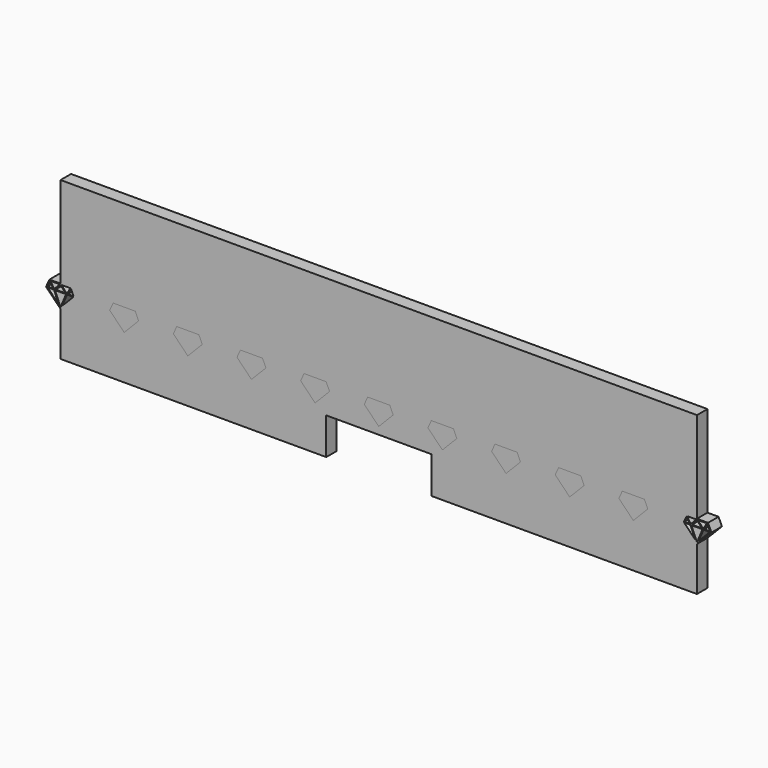
from build123d import *

# Parameters (mm, degrees)
F2_DEPTH = 1.6
F5_DEPTH = 25


# Not quite as in the source:
# - a feature of the source that left no trace in its solid (it failed there, or was rolled back) is left out
# - a feature names something its author has since deleted; it is built from what else it names


with BuildPart() as f2:
    # F0 (on Front) → F2 (new body)
    with BuildSketch(Plane.XZ):
        Polygon((-27.5092766582, 112.0762870512), (0, 83.9119844419), (27.5092766582, 112.0762870512), (21.0788567191, 126.3461877986), (0, 126.3459026814), (-21.0788567191, 126.3461877986), align=None)
        Polygon((-24.595520188, 111.955450038), (-12.439796289, 111.955450038), (-3.5350198746, 90.3934761882), align=None, mode=Mode.SUBTRACT)
        Polygon((10.5240828187, 111.955450038), (0, 86.5410715342), (-10.5240828187, 111.955450038), (0, 111.955450038), align=None, mode=Mode.SUBTRACT)
        Polygon((24.595520188, 111.955450038), (3.5350198746, 90.3934761882), (12.439796289, 111.955450038), align=None, mode=Mode.SUBTRACT)
        Polygon((-19.8720569611, 124.1561621428), (-13.9740581512, 113.2946610451), (-24.7665558411, 113.2946610451), align=None, mode=Mode.SUBTRACT)
        Polygon((-18.6457509995, 124.6817186475), (-1.7468536503, 124.6817186475), (-12.1264214497, 113.0322592129), align=None, mode=Mode.SUBTRACT)
        Polygon((-9.4357720005, 113.2946610451), (0, 123.8848556735), (9.4357720005, 113.2946610451), (0, 113.2946610451), align=None, mode=Mode.SUBTRACT)
        Polygon((12.1264214497, 113.0322592129), (1.7468536503, 124.6817186475), (18.6457509995, 124.6817186475), align=None, mode=Mode.SUBTRACT)
        Polygon((13.9740581512, 113.2946610451), (19.8720569611, 124.1561621428), (24.7665558411, 113.2946610451), align=None, mode=Mode.SUBTRACT)
    extrude(amount=-F2_DEPTH)


with BuildPart() as f2b:
    # F0 (on Front) → F2, piece 2 (new body)
    with BuildSketch(Plane.XZ):
        Polygon((-1069.7211432809, 126.3461877986), (-1090.8, 126.3459026814), (-1111.8788567191, 126.3461877986), (-1118.3092766582, 112.0762870511), (-1090.8, 83.9119844419), (-1063.2907233418, 112.0762870512), align=None)
        Polygon((-1115.395520188, 111.955450038), (-1103.239796289, 111.955450038), (-1094.3350198746, 90.3934761882), align=None, mode=Mode.SUBTRACT)
        Polygon((-1080.2759171813, 111.955450038), (-1090.8, 86.5410715342), (-1101.3240828187, 111.955450038), (-1090.8, 111.955450038), align=None, mode=Mode.SUBTRACT)
        Polygon((-1066.204479812, 111.955450038), (-1087.2649801254, 90.3934761882), (-1078.360203711, 111.955450038), align=None, mode=Mode.SUBTRACT)
        Polygon((-1110.6720569611, 124.1561621428), (-1104.7740581512, 113.2946610451), (-1115.5665558411, 113.2946610451), align=None, mode=Mode.SUBTRACT)
        Polygon((-1109.4457509995, 124.6817186475), (-1092.5468536503, 124.6817186475), (-1102.9264214497, 113.0322592129), align=None, mode=Mode.SUBTRACT)
        Polygon((-1100.2357720005, 113.2946610451), (-1090.8, 123.8848556735), (-1081.3642279995, 113.2946610451), (-1090.8, 113.2946610451), align=None, mode=Mode.SUBTRACT)
        Polygon((-1078.6735785503, 113.0322592129), (-1089.0531463497, 124.6817186475), (-1072.1542490005, 124.6817186475), align=None, mode=Mode.SUBTRACT)
        Polygon((-1076.8259418488, 113.2946610451), (-1070.9279430389, 124.1561621428), (-1066.0334441589, 113.2946610451), align=None, mode=Mode.SUBTRACT)
        Polygon((-1081.3642279995, 113.2946610451), (-1090.8, 123.8848556735), (-1100.2357720005, 113.2946610451), (-1090.8, 113.2946610451), align=None)
        Polygon((-1102.9264214497, 113.0322592129), (-1092.5468536503, 124.6817186475), (-1109.4457509995, 124.6817186475), align=None)
        Polygon((-1072.1542490005, 124.6817186475), (-1089.0531463497, 124.6817186475), (-1078.6735785503, 113.0322592129), align=None)
        Polygon((-1066.0334441589, 113.2946610451), (-1070.9279430389, 124.1561621428), (-1076.8259418488, 113.2946610451), align=None)
        Polygon((-1078.360203711, 111.955450038), (-1087.2649801254, 90.3934761882), (-1066.204479812, 111.955450038), align=None)
        Polygon((-1101.3240828187, 111.955450038), (-1090.8, 86.5410715342), (-1080.2759171813, 111.955450038), (-1090.8, 111.955450038), align=None)
        Polygon((-1094.3350198746, 90.3934761882), (-1103.239796289, 111.955450038), (-1115.395520188, 111.955450038), align=None)
        Polygon((-1115.5665558411, 113.2946610451), (-1104.7740581512, 113.2946610451), (-1110.6720569611, 124.1561621428), align=None)
    extrude(amount=-F2_DEPTH)


with BuildPart() as f2c:
    # F0 (on Front) → F2, piece 3 (new body)
    with BuildSketch(Plane.XZ):
        Polygon((-948.5211432809, 126.3461877986), (-969.6, 126.3459026814), (-990.6788567191, 126.3461877986), (-997.1092766582, 112.0762870511), (-969.6, 83.9119844419), (-942.0907233418, 112.0762870512), align=None)
        Polygon((-994.195520188, 111.955450038), (-982.039796289, 111.955450038), (-973.1350198746, 90.3934761882), align=None, mode=Mode.SUBTRACT)
        Polygon((-959.0759171813, 111.955450038), (-969.6, 86.5410715342), (-980.1240828187, 111.955450038), (-969.6, 111.955450038), align=None, mode=Mode.SUBTRACT)
        Polygon((-945.004479812, 111.955450038), (-966.0649801254, 90.3934761882), (-957.160203711, 111.955450038), align=None, mode=Mode.SUBTRACT)
        Polygon((-989.4720569611, 124.1561621428), (-983.5740581512, 113.2946610451), (-994.3665558411, 113.2946610451), align=None, mode=Mode.SUBTRACT)
        Polygon((-988.2457509995, 124.6817186475), (-971.3468536503, 124.6817186475), (-981.7264214497, 113.0322592129), align=None, mode=Mode.SUBTRACT)
        Polygon((-979.0357720005, 113.2946610451), (-969.6, 123.8848556735), (-960.1642279995, 113.2946610451), (-969.6, 113.2946610451), align=None, mode=Mode.SUBTRACT)
        Polygon((-957.4735785503, 113.0322592129), (-967.8531463497, 124.6817186475), (-950.9542490005, 124.6817186475), align=None, mode=Mode.SUBTRACT)
        Polygon((-955.6259418488, 113.2946610451), (-949.7279430389, 124.1561621428), (-944.8334441589, 113.2946610451), align=None, mode=Mode.SUBTRACT)
        Polygon((-960.1642279995, 113.2946610451), (-969.6, 123.8848556735), (-979.0357720005, 113.2946610451), (-969.6, 113.2946610451), align=None)
        Polygon((-981.7264214497, 113.0322592129), (-971.3468536503, 124.6817186475), (-988.2457509995, 124.6817186475), align=None)
        Polygon((-950.9542490005, 124.6817186475), (-967.8531463497, 124.6817186475), (-957.4735785503, 113.0322592129), align=None)
        Polygon((-944.8334441589, 113.2946610451), (-949.7279430389, 124.1561621428), (-955.6259418488, 113.2946610451), align=None)
        Polygon((-957.160203711, 111.955450038), (-966.0649801254, 90.3934761882), (-945.004479812, 111.955450038), align=None)
        Polygon((-980.1240828187, 111.955450038), (-969.6, 86.5410715342), (-959.0759171813, 111.955450038), (-969.6, 111.955450038), align=None)
        Polygon((-973.1350198746, 90.3934761882), (-982.039796289, 111.955450038), (-994.195520188, 111.955450038), align=None)
        Polygon((-994.3665558411, 113.2946610451), (-983.5740581512, 113.2946610451), (-989.4720569611, 124.1561621428), align=None)
    extrude(amount=-F2_DEPTH)


with BuildPart() as f2d:
    # F0 (on Front) → F2, piece 4 (new body)
    with BuildSketch(Plane.XZ):
        Polygon((-827.3211432809, 126.3461877986), (-848.4, 126.3459026814), (-869.4788567191, 126.3461877986), (-875.9092766582, 112.0762870511), (-848.4, 83.9119844419), (-820.8907233418, 112.0762870512), align=None)
        Polygon((-837.8759171813, 111.955450038), (-848.4, 86.5410715342), (-858.9240828187, 111.955450038), (-848.4, 111.955450038), align=None, mode=Mode.SUBTRACT)
        Polygon((-872.995520188, 111.955450038), (-860.839796289, 111.955450038), (-851.9350198746, 90.3934761882), align=None, mode=Mode.SUBTRACT)
        Polygon((-823.804479812, 111.955450038), (-844.8649801254, 90.3934761882), (-835.960203711, 111.955450038), align=None, mode=Mode.SUBTRACT)
        Polygon((-868.2720569611, 124.1561621428), (-862.3740581512, 113.2946610451), (-873.1665558411, 113.2946610451), align=None, mode=Mode.SUBTRACT)
        Polygon((-867.0457509995, 124.6817186475), (-850.1468536503, 124.6817186475), (-860.5264214497, 113.0322592129), align=None, mode=Mode.SUBTRACT)
        Polygon((-857.8357720005, 113.2946610451), (-848.4, 123.8848556735), (-838.9642279995, 113.2946610451), (-848.4, 113.2946610451), align=None, mode=Mode.SUBTRACT)
        Polygon((-836.2735785503, 113.0322592129), (-846.6531463497, 124.6817186475), (-829.7542490005, 124.6817186475), align=None, mode=Mode.SUBTRACT)
        Polygon((-838.9642279995, 113.2946610451), (-848.4, 123.8848556735), (-857.8357720005, 113.2946610451), (-848.4, 113.2946610451), align=None)
        Polygon((-860.5264214497, 113.0322592129), (-850.1468536503, 124.6817186475), (-867.0457509995, 124.6817186475), align=None)
        Polygon((-829.7542490005, 124.6817186475), (-846.6531463497, 124.6817186475), (-836.2735785503, 113.0322592129), align=None)
        Polygon((-835.960203711, 111.955450038), (-844.8649801254, 90.3934761882), (-823.804479812, 111.955450038), align=None)
        Polygon((-858.9240828187, 111.955450038), (-848.4, 86.5410715342), (-837.8759171813, 111.955450038), (-848.4, 111.955450038), align=None)
        Polygon((-851.9350198746, 90.3934761882), (-860.839796289, 111.955450038), (-872.995520188, 111.955450038), align=None)
        Polygon((-873.1665558411, 113.2946610451), (-862.3740581512, 113.2946610451), (-868.2720569611, 124.1561621428), align=None)
    extrude(amount=-F2_DEPTH)


with BuildPart() as f2e:
    # F0 (on Front) → F2, piece 5 (new body)
    with BuildSketch(Plane.XZ):
        Polygon((-706.1211432809, 126.3461877986), (-727.2, 126.3459026814), (-748.2788567191, 126.3461877986), (-754.7092766582, 112.0762870511), (-727.2, 83.9119844419), (-699.6907233418, 112.0762870512), align=None)
        Polygon((-716.6759171813, 111.955450038), (-727.2, 86.5410715342), (-737.7240828187, 111.955450038), (-727.2, 111.955450038), align=None, mode=Mode.SUBTRACT)
        Polygon((-751.795520188, 111.955450038), (-739.639796289, 111.955450038), (-730.7350198746, 90.3934761882), align=None, mode=Mode.SUBTRACT)
        Polygon((-702.604479812, 111.955450038), (-723.6649801254, 90.3934761882), (-714.760203711, 111.955450038), align=None, mode=Mode.SUBTRACT)
        Polygon((-747.0720569611, 124.1561621428), (-741.1740581512, 113.2946610451), (-751.9665558411, 113.2946610451), align=None, mode=Mode.SUBTRACT)
        Polygon((-745.8457509995, 124.6817186475), (-728.9468536503, 124.6817186475), (-739.3264214497, 113.0322592129), align=None, mode=Mode.SUBTRACT)
        Polygon((-736.6357720005, 113.2946610451), (-727.2, 123.8848556735), (-717.7642279995, 113.2946610451), (-727.2, 113.2946610451), align=None, mode=Mode.SUBTRACT)
        Polygon((-715.0735785503, 113.0322592129), (-725.4531463497, 124.6817186475), (-708.5542490005, 124.6817186475), align=None, mode=Mode.SUBTRACT)
        Polygon((-717.7642279995, 113.2946610451), (-727.2, 123.8848556735), (-736.6357720005, 113.2946610451), (-727.2, 113.2946610451), align=None)
        Polygon((-739.3264214497, 113.0322592129), (-728.9468536503, 124.6817186475), (-745.8457509995, 124.6817186475), align=None)
        Polygon((-708.5542490005, 124.6817186475), (-725.4531463497, 124.6817186475), (-715.0735785503, 113.0322592129), align=None)
        Polygon((-714.760203711, 111.955450038), (-723.6649801254, 90.3934761882), (-702.604479812, 111.955450038), align=None)
        Polygon((-737.7240828187, 111.955450038), (-727.2, 86.5410715342), (-716.6759171813, 111.955450038), (-727.2, 111.955450038), align=None)
        Polygon((-730.7350198746, 90.3934761882), (-739.639796289, 111.955450038), (-751.795520188, 111.955450038), align=None)
        Polygon((-751.9665558411, 113.2946610451), (-741.1740581512, 113.2946610451), (-747.0720569611, 124.1561621428), align=None)
    extrude(amount=-F2_DEPTH)


with BuildPart() as f2f:
    # F0 (on Front) → F2, piece 6 (new body)
    with BuildSketch(Plane.XZ):
        Polygon((-584.9211432809, 126.3461877986), (-606, 126.3459026814), (-627.0788567191, 126.3461877986), (-633.5092766582, 112.0762870511), (-606, 83.9119844419), (-578.4907233418, 112.0762870512), align=None)
        Polygon((-630.595520188, 111.955450038), (-618.439796289, 111.955450038), (-609.5350198746, 90.3934761882), align=None, mode=Mode.SUBTRACT)
        Polygon((-625.8720569611, 124.1561621428), (-619.9740581512, 113.2946610451), (-630.7665558411, 113.2946610451), align=None, mode=Mode.SUBTRACT)
        Polygon((-624.6457509995, 124.6817186475), (-607.7468536503, 124.6817186475), (-618.1264214497, 113.0322592129), align=None, mode=Mode.SUBTRACT)
        Polygon((-595.4759171813, 111.955450038), (-606, 86.5410715342), (-616.5240828187, 111.955450038), (-606, 111.955450038), align=None, mode=Mode.SUBTRACT)
        Polygon((-581.404479812, 111.955450038), (-602.4649801254, 90.3934761882), (-593.560203711, 111.955450038), align=None, mode=Mode.SUBTRACT)
        Polygon((-615.4357720005, 113.2946610451), (-606, 123.8848556735), (-596.5642279995, 113.2946610451), (-606, 113.2946610451), align=None, mode=Mode.SUBTRACT)
        Polygon((-593.8735785503, 113.0322592129), (-604.2531463497, 124.6817186475), (-587.3542490005, 124.6817186475), align=None, mode=Mode.SUBTRACT)
        Polygon((-596.5642279995, 113.2946610451), (-606, 123.8848556735), (-615.4357720005, 113.2946610451), (-606, 113.2946610451), align=None)
        Polygon((-618.1264214497, 113.0322592129), (-607.7468536503, 124.6817186475), (-624.6457509995, 124.6817186475), align=None)
        Polygon((-587.3542490005, 124.6817186475), (-604.2531463497, 124.6817186475), (-593.8735785503, 113.0322592129), align=None)
        Polygon((-593.560203711, 111.955450038), (-602.4649801254, 90.3934761882), (-581.404479812, 111.955450038), align=None)
        Polygon((-616.5240828187, 111.955450038), (-606, 86.5410715342), (-595.4759171813, 111.955450038), (-606, 111.955450038), align=None)
        Polygon((-609.5350198746, 90.3934761882), (-618.439796289, 111.955450038), (-630.595520188, 111.955450038), align=None)
        Polygon((-630.7665558411, 113.2946610451), (-619.9740581512, 113.2946610451), (-625.8720569611, 124.1561621428), align=None)
    extrude(amount=-F2_DEPTH)


with BuildPart() as f2g:
    # F0 (on Front) → F2, piece 7 (new body)
    with BuildSketch(Plane.XZ):
        Polygon((-463.7211432809, 126.3461877986), (-484.8, 126.3459026814), (-505.8788567191, 126.3461877986), (-512.3092766582, 112.0762870511), (-484.8, 83.9119844419), (-457.2907233418, 112.0762870512), align=None)
        Polygon((-509.395520188, 111.955450038), (-497.239796289, 111.955450038), (-488.3350198746, 90.3934761882), align=None, mode=Mode.SUBTRACT)
        Polygon((-474.2759171813, 111.955450038), (-484.8, 86.5410715342), (-495.3240828187, 111.955450038), (-484.8, 111.955450038), align=None, mode=Mode.SUBTRACT)
        Polygon((-460.204479812, 111.955450038), (-481.2649801254, 90.3934761882), (-472.360203711, 111.955450038), align=None, mode=Mode.SUBTRACT)
        Polygon((-504.6720569611, 124.1561621428), (-498.7740581512, 113.2946610451), (-509.5665558411, 113.2946610451), align=None, mode=Mode.SUBTRACT)
        Polygon((-503.4457509995, 124.6817186475), (-486.5468536503, 124.6817186475), (-496.9264214497, 113.0322592129), align=None, mode=Mode.SUBTRACT)
        Polygon((-494.2357720005, 113.2946610451), (-484.8, 123.8848556735), (-475.3642279995, 113.2946610451), (-484.8, 113.2946610451), align=None, mode=Mode.SUBTRACT)
        Polygon((-472.6735785503, 113.0322592129), (-483.0531463497, 124.6817186475), (-466.1542490005, 124.6817186475), align=None, mode=Mode.SUBTRACT)
        Polygon((-475.3642279995, 113.2946610451), (-484.8, 123.8848556735), (-494.2357720005, 113.2946610451), (-484.8, 113.2946610451), align=None)
        Polygon((-496.9264214497, 113.0322592129), (-486.5468536503, 124.6817186475), (-503.4457509995, 124.6817186475), align=None)
        Polygon((-466.1542490005, 124.6817186475), (-483.0531463497, 124.6817186475), (-472.6735785503, 113.0322592129), align=None)
        Polygon((-472.360203711, 111.955450038), (-481.2649801254, 90.3934761882), (-460.204479812, 111.955450038), align=None)
        Polygon((-495.3240828187, 111.955450038), (-484.8, 86.5410715342), (-474.2759171813, 111.955450038), (-484.8, 111.955450038), align=None)
        Polygon((-488.3350198746, 90.3934761882), (-497.239796289, 111.955450038), (-509.395520188, 111.955450038), align=None)
        Polygon((-509.5665558411, 113.2946610451), (-498.7740581512, 113.2946610451), (-504.6720569611, 124.1561621428), align=None)
    extrude(amount=-F2_DEPTH)


with BuildPart() as f2h:
    # F0 (on Front) → F2, piece 8 (new body)
    with BuildSketch(Plane.XZ):
        Polygon((-342.5211432809, 126.3461877986), (-363.6, 126.3459026814), (-384.6788567191, 126.3461877986), (-391.1092766582, 112.0762870511), (-363.6, 83.9119844419), (-336.0907233418, 112.0762870512), align=None)
        Polygon((-388.195520188, 111.955450038), (-376.039796289, 111.955450038), (-367.1350198746, 90.3934761882), align=None, mode=Mode.SUBTRACT)
        Polygon((-353.0759171813, 111.955450038), (-363.6, 86.5410715342), (-374.1240828187, 111.955450038), (-363.6, 111.955450038), align=None, mode=Mode.SUBTRACT)
        Polygon((-339.004479812, 111.955450038), (-360.0649801254, 90.3934761882), (-351.160203711, 111.955450038), align=None, mode=Mode.SUBTRACT)
        Polygon((-383.4720569611, 124.1561621428), (-377.5740581512, 113.2946610451), (-388.3665558411, 113.2946610451), align=None, mode=Mode.SUBTRACT)
        Polygon((-382.2457509995, 124.6817186475), (-365.3468536503, 124.6817186475), (-375.7264214497, 113.0322592129), align=None, mode=Mode.SUBTRACT)
        Polygon((-373.0357720005, 113.2946610451), (-363.6, 123.8848556735), (-354.1642279995, 113.2946610451), (-363.6, 113.2946610451), align=None, mode=Mode.SUBTRACT)
        Polygon((-351.4735785503, 113.0322592129), (-361.8531463497, 124.6817186475), (-344.9542490005, 124.6817186475), align=None, mode=Mode.SUBTRACT)
        Polygon((-354.1642279995, 113.2946610451), (-363.6, 123.8848556735), (-373.0357720005, 113.2946610451), (-363.6, 113.2946610451), align=None)
        Polygon((-375.7264214497, 113.0322592129), (-365.3468536503, 124.6817186475), (-382.2457509995, 124.6817186475), align=None)
        Polygon((-344.9542490005, 124.6817186475), (-361.8531463497, 124.6817186475), (-351.4735785503, 113.0322592129), align=None)
        Polygon((-351.160203711, 111.955450038), (-360.0649801254, 90.3934761882), (-339.004479812, 111.955450038), align=None)
        Polygon((-374.1240828187, 111.955450038), (-363.6, 86.5410715342), (-353.0759171813, 111.955450038), (-363.6, 111.955450038), align=None)
        Polygon((-367.1350198746, 90.3934761882), (-376.039796289, 111.955450038), (-388.195520188, 111.955450038), align=None)
        Polygon((-388.3665558411, 113.2946610451), (-377.5740581512, 113.2946610451), (-383.4720569611, 124.1561621428), align=None)
    extrude(amount=-F2_DEPTH)


with BuildPart() as f2i:
    # F0 (on Front) → F2, piece 9 (new body)
    with BuildSketch(Plane.XZ):
        Polygon((-221.3211432809, 126.3461877986), (-242.4, 126.3459026814), (-263.4788567191, 126.3461877986), (-269.9092766582, 112.0762870511), (-242.4, 83.9119844419), (-214.8907233418, 112.0762870512), align=None)
        Polygon((-266.995520188, 111.955450038), (-254.839796289, 111.955450038), (-245.9350198746, 90.3934761882), align=None, mode=Mode.SUBTRACT)
        Polygon((-231.8759171813, 111.955450038), (-242.4, 86.5410715342), (-252.9240828187, 111.955450038), (-242.4, 111.955450038), align=None, mode=Mode.SUBTRACT)
        Polygon((-217.804479812, 111.955450038), (-238.8649801254, 90.3934761882), (-229.960203711, 111.955450038), align=None, mode=Mode.SUBTRACT)
        Polygon((-262.2720569611, 124.1561621428), (-256.3740581512, 113.2946610451), (-267.1665558411, 113.2946610451), align=None, mode=Mode.SUBTRACT)
        Polygon((-261.0457509995, 124.6817186475), (-244.1468536503, 124.6817186475), (-254.5264214497, 113.0322592129), align=None, mode=Mode.SUBTRACT)
        Polygon((-251.8357720005, 113.2946610451), (-242.4, 123.8848556735), (-232.9642279995, 113.2946610451), (-242.4, 113.2946610451), align=None, mode=Mode.SUBTRACT)
        Polygon((-230.2735785503, 113.0322592129), (-240.6531463497, 124.6817186475), (-223.7542490005, 124.6817186475), align=None, mode=Mode.SUBTRACT)
        Polygon((-232.9642279995, 113.2946610451), (-242.4, 123.8848556735), (-251.8357720005, 113.2946610451), (-242.4, 113.2946610451), align=None)
        Polygon((-254.5264214497, 113.0322592129), (-244.1468536503, 124.6817186475), (-261.0457509995, 124.6817186475), align=None)
        Polygon((-223.7542490005, 124.6817186475), (-240.6531463497, 124.6817186475), (-230.2735785503, 113.0322592129), align=None)
        Polygon((-229.960203711, 111.955450038), (-238.8649801254, 90.3934761882), (-217.804479812, 111.955450038), align=None)
        Polygon((-252.9240828187, 111.955450038), (-242.4, 86.5410715342), (-231.8759171813, 111.955450038), (-242.4, 111.955450038), align=None)
        Polygon((-245.9350198746, 90.3934761882), (-254.839796289, 111.955450038), (-266.995520188, 111.955450038), align=None)
        Polygon((-267.1665558411, 113.2946610451), (-256.3740581512, 113.2946610451), (-262.2720569611, 124.1561621428), align=None)
    extrude(amount=-F2_DEPTH)


with BuildPart() as f2j:
    # F0 (on Front) → F2, piece 10 (new body)
    with BuildSketch(Plane.XZ):
        Polygon((-100.1211432809, 126.3461877986), (-121.2, 126.3459026814), (-142.2788567191, 126.3461877986), (-148.7092766582, 112.0762870511), (-121.2, 83.9119844419), (-93.6907233418, 112.0762870512), align=None)
        Polygon((-145.795520188, 111.955450038), (-133.639796289, 111.955450038), (-124.7350198746, 90.3934761882), align=None, mode=Mode.SUBTRACT)
        Polygon((-110.6759171813, 111.955450038), (-121.2, 86.5410715342), (-131.7240828187, 111.955450038), (-121.2, 111.955450038), align=None, mode=Mode.SUBTRACT)
        Polygon((-96.604479812, 111.955450038), (-117.6649801254, 90.3934761882), (-108.760203711, 111.955450038), align=None, mode=Mode.SUBTRACT)
        Polygon((-141.0720569611, 124.1561621428), (-135.1740581512, 113.2946610451), (-145.9665558411, 113.2946610451), align=None, mode=Mode.SUBTRACT)
        Polygon((-139.8457509995, 124.6817186475), (-122.9468536503, 124.6817186475), (-133.3264214497, 113.0322592129), align=None, mode=Mode.SUBTRACT)
        Polygon((-130.6357720005, 113.2946610451), (-121.2, 123.8848556735), (-111.7642279995, 113.2946610451), (-121.2, 113.2946610451), align=None, mode=Mode.SUBTRACT)
        Polygon((-109.0735785503, 113.0322592129), (-119.4531463497, 124.6817186475), (-102.5542490005, 124.6817186475), align=None, mode=Mode.SUBTRACT)
        Polygon((-111.7642279995, 113.2946610451), (-121.2, 123.8848556735), (-130.6357720005, 113.2946610451), (-121.2, 113.2946610451), align=None)
        Polygon((-133.3264214497, 113.0322592129), (-122.9468536503, 124.6817186475), (-139.8457509995, 124.6817186475), align=None)
        Polygon((-102.5542490005, 124.6817186475), (-119.4531463497, 124.6817186475), (-109.0735785503, 113.0322592129), align=None)
        Polygon((-108.760203711, 111.955450038), (-117.6649801254, 90.3934761882), (-96.604479812, 111.955450038), align=None)
        Polygon((-131.7240828187, 111.955450038), (-121.2, 86.5410715342), (-110.6759171813, 111.955450038), (-121.2, 111.955450038), align=None)
        Polygon((-124.7350198746, 90.3934761882), (-133.639796289, 111.955450038), (-145.795520188, 111.955450038), align=None)
        Polygon((-145.9665558411, 113.2946610451), (-135.1740581512, 113.2946610451), (-141.0720569611, 124.1561621428), align=None)
    extrude(amount=-F2_DEPTH)


with BuildPart() as f5:
    # F0 (on Front) → F5 (new body)
    with BuildSketch(Plane.XZ):
        Polygon((-506, 0), (0, 0), (0, 83.9119844419), (-27.5092766582, 112.0762870512), (-21.0788567191, 126.3461877986), (0, 126.3459026814), (0, 139.5855637093), (0, 300), (-1212, 300), (-1212, 139.5855637093), (-1212, 126.3459026814), (-1190.9211432809, 126.3461877986), (-1184.4907233418, 112.0762870511), (-1212, 83.9119844419), (-1212, 0), (-706, 0), (-706, 70), (-506, 70), align=None)
        Polygon((-1111.8788567191, 126.3461877986), (-1090.8, 126.3459026814), (-1069.7211432809, 126.3461877986), (-1063.2907233418, 112.0762870511), (-1090.8, 83.9119844419), (-1118.3092766582, 112.0762870512), align=None, mode=Mode.SUBTRACT)
        Polygon((-990.6788567191, 126.3461877986), (-969.6, 126.3459026814), (-948.5211432809, 126.3461877986), (-942.0907233418, 112.0762870511), (-969.6, 83.9119844419), (-997.1092766582, 112.0762870512), align=None, mode=Mode.SUBTRACT)
        Polygon((-869.4788567191, 126.3461877986), (-848.4, 126.3459026814), (-827.3211432809, 126.3461877986), (-820.8907233418, 112.0762870511), (-848.4, 83.9119844419), (-875.9092766582, 112.0762870512), align=None, mode=Mode.SUBTRACT)
        Polygon((-748.2788567191, 126.3461877986), (-727.2, 126.3459026814), (-706.1211432809, 126.3461877986), (-699.6907233418, 112.0762870511), (-727.2, 83.9119844419), (-754.7092766582, 112.0762870512), align=None, mode=Mode.SUBTRACT)
        Polygon((-627.0788567191, 126.3461877986), (-606, 126.3459026814), (-584.9211432809, 126.3461877986), (-578.4907233418, 112.0762870511), (-606, 83.9119844419), (-633.5092766582, 112.0762870512), align=None, mode=Mode.SUBTRACT)
        Polygon((-505.8788567191, 126.3461877986), (-484.8, 126.3459026814), (-463.7211432809, 126.3461877986), (-457.2907233418, 112.0762870511), (-484.8, 83.9119844419), (-512.3092766582, 112.0762870512), align=None, mode=Mode.SUBTRACT)
        Polygon((-384.6788567191, 126.3461877986), (-363.6, 126.3459026814), (-342.5211432809, 126.3461877986), (-336.0907233418, 112.0762870511), (-363.6, 83.9119844419), (-391.1092766582, 112.0762870512), align=None, mode=Mode.SUBTRACT)
        Polygon((-263.4788567191, 126.3461877986), (-242.4, 126.3459026814), (-221.3211432809, 126.3461877986), (-214.8907233418, 112.0762870511), (-242.4, 83.9119844419), (-269.9092766582, 112.0762870512), align=None, mode=Mode.SUBTRACT)
        Polygon((-142.2788567191, 126.3461877986), (-121.2, 126.3459026814), (-100.1211432809, 126.3461877986), (-93.6907233418, 112.0762870511), (-121.2, 83.9119844419), (-148.7092766582, 112.0762870512), align=None, mode=Mode.SUBTRACT)
        Polygon((-27.5092766582, 112.0762870512), (0, 83.9119844419), (27.5092766582, 112.0762870512), (21.0788567191, 126.3461877986), (0, 126.3459026814), (-21.0788567191, 126.3461877986), align=None)
        Polygon((-24.595520188, 111.955450038), (-12.439796289, 111.955450038), (-3.5350198746, 90.3934761882), align=None, mode=Mode.SUBTRACT)
        Polygon((10.5240828187, 111.955450038), (0, 86.5410715342), (-10.5240828187, 111.955450038), (0, 111.955450038), align=None, mode=Mode.SUBTRACT)
        Polygon((24.595520188, 111.955450038), (3.5350198746, 90.3934761882), (12.439796289, 111.955450038), align=None, mode=Mode.SUBTRACT)
        Polygon((-19.8720569611, 124.1561621428), (-13.9740581512, 113.2946610451), (-24.7665558411, 113.2946610451), align=None, mode=Mode.SUBTRACT)
        Polygon((-18.6457509995, 124.6817186475), (-1.7468536503, 124.6817186475), (-12.1264214497, 113.0322592129), align=None, mode=Mode.SUBTRACT)
        Polygon((-9.4357720005, 113.2946610451), (0, 123.8848556735), (9.4357720005, 113.2946610451), (0, 113.2946610451), align=None, mode=Mode.SUBTRACT)
        Polygon((12.1264214497, 113.0322592129), (1.7468536503, 124.6817186475), (18.6457509995, 124.6817186475), align=None, mode=Mode.SUBTRACT)
        Polygon((13.9740581512, 113.2946610451), (19.8720569611, 124.1561621428), (24.7665558411, 113.2946610451), align=None, mode=Mode.SUBTRACT)
        Polygon((-1239.5092766582, 112.0762870512), (-1212, 83.9119844419), (-1184.4907233418, 112.0762870512), (-1190.9211432809, 126.3461877986), (-1212, 126.3459026814), (-1233.0788567191, 126.3461877986), align=None)
        Polygon((-1215.5350198746, 90.3934761882), (-1236.595520188, 111.955450038), (-1224.439796289, 111.955450038), align=None, mode=Mode.SUBTRACT)
        Polygon((-1201.4759171813, 111.955450038), (-1212, 86.5410715342), (-1222.5240828187, 111.955450038), (-1212, 111.955450038), align=None, mode=Mode.SUBTRACT)
        Polygon((-1208.4649801254, 90.3934761882), (-1199.560203711, 111.955450038), (-1187.404479812, 111.955450038), align=None, mode=Mode.SUBTRACT)
        Polygon((-1236.7665558411, 113.2946610451), (-1231.8720569611, 124.1561621428), (-1225.9740581512, 113.2946610451), align=None, mode=Mode.SUBTRACT)
        Polygon((-1224.1264214497, 113.0322592129), (-1230.6457509995, 124.6817186475), (-1213.7468536503, 124.6817186475), align=None, mode=Mode.SUBTRACT)
        Polygon((-1202.5642279995, 113.2946610451), (-1212, 113.2946610451), (-1221.4357720005, 113.2946610451), (-1212, 123.8848556735), align=None, mode=Mode.SUBTRACT)
        Polygon((-1199.8735785503, 113.0322592129), (-1210.2531463497, 124.6817186475), (-1193.3542490005, 124.6817186475), align=None, mode=Mode.SUBTRACT)
        Polygon((-1187.2334441589, 113.2946610451), (-1198.0259418488, 113.2946610451), (-1192.1279430389, 124.1561621428), align=None, mode=Mode.SUBTRACT)
    extrude(amount=-F5_DEPTH)


solid = Compound([f2.part, f2b.part, f2c.part, f2d.part, f2e.part, f2f.part, f2g.part, f2h.part, f2i.part, f2j.part, f5.part])
